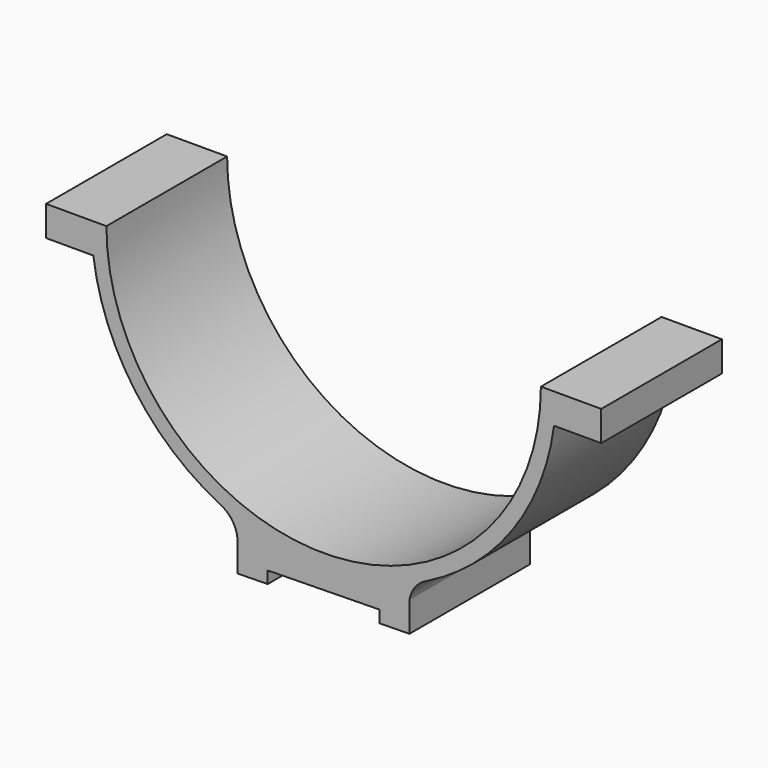
from build123d import *

# Parameters (mm, degrees)
F1_DEPTH    = 25
F2_T1_DEPTH = 25


# Not quite as in the source:
# - a fillet or chamfer that OpenCascade refuses, or shapes differently, is made with other operations: its cross-section is extruded or revolved along the edge and cut away or added


with BuildPart() as f1:
    # F0 (on Front) → F1 (new body)
    with BuildSketch(Plane.XZ):
        with BuildLine():
            ThreePointArc((36, 0), (0, -36), (-36, 0))
            Line((-36, 0), (-38.5, 0))
            Line((-38.5, 0), (-46, 0))
            Line((-46, 0), (-46, -5))
            Line((-46, -5), (-38.1739439933, -5))
            ThreePointArc((-38.1739439933, -5), (-26.2977937101, -28.1189623916), (-2.4365316343, -38.4228228218))
            Line((-2.4365316343, -38.4228228218), (-14.2752447595, -38.6175373625))
            Line((-14.2752447595, -38.6175373625), (-14.2752447595, -43.6175822914))
            Line((-14.2752447595, -43.6175822914), (-9.2752447595, -43.5353459289))
            Line((-9.2752447595, -43.5353459289), (-9.2752447595, -41.5353459289))
            Line((-9.2752447595, -41.5353459289), (9.222253505, -41.2311125346))
            Line((9.222253505, -41.2311125346), (9.222253505, -43.2311125346))
            Line((9.222253505, -43.2311125346), (14.222253505, -43.1488761722))
            Line((14.222253505, -43.1488761722), (14.222253505, -38.1488312433))
            Line((14.222253505, -38.1488312433), (3.6987732294, -38.3219137909))
            ThreePointArc((3.6987732294, -38.3219137909), (26.7566551829, -27.682691405), (38.1739439933, -5))
            Line((38.1739439933, -5), (46, -5))
            Line((46, -5), (46, 0))
            Line((46, 0), (38.5, 0))
            Line((38.5, 0), (36, 0))
        make_face()
    extrude(amount=F1_DEPTH)

    # F2: fillet of radius 5 on 2 edges, made by hand

    # F2_s2 → F2_t1 (join)
    with BuildSketch(Plane.XZ):
        with BuildLine():
            ThreePointArc((-14.2752447595, -38.6175373625), (-15.118767178, -36.2023611517), (-17.0464798519, -34.5205377226))
            ThreePointArc((-17.0464798519, -34.5205377226), (-9.9349832104, -37.1960496371), (-2.4365316343, -38.4228228218))
            Line((-2.4365316343, -38.4228228218), (-14.2752447595, -38.6175373625))
        make_face()
        with BuildLine():
            ThreePointArc((16.9380433228, -34.5738729158), (15.1563460299, -36.0394019773), (14.222253505, -38.1488312433))
            Line((14.222253505, -38.1488312433), (3.6987732294, -38.3219137909))
            ThreePointArc((3.6987732294, -38.3219137909), (10.4872065848, -37.0441425606), (16.9380433228, -34.5738729158))
        make_face()
    extrude(amount=F2_T1_DEPTH)


solid = f1.part
